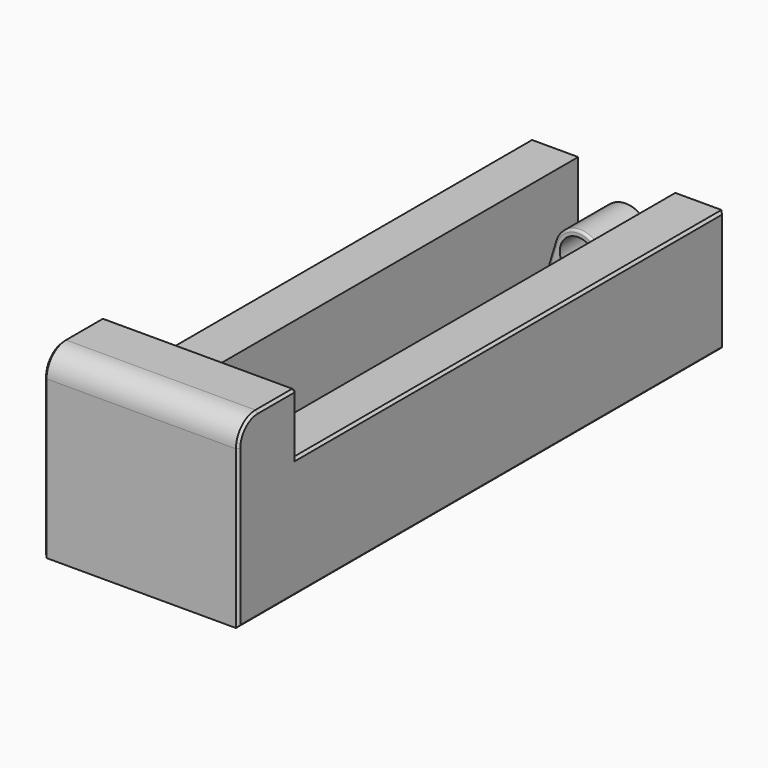
from build123d import *

# Parameters (mm, degrees)
F1_DEPTH = 40
F2_R     = 7.6
F3_DEPTH = 220
F4_DEPTH = 25
F5_SIZE  = 1
F6_R     = 1


with BuildPart() as f1:
    # F0 (on Right) → F1 (new body, symmetric)
    with BuildSketch(Plane.YZ):
        with BuildLine():
            Line((-146.159631235, 0), (0, 0))
            Line((0, 0), (45.9261649855, 0))
            Line((45.9261649855, 0), (103.840368765, 0))
            Line((103.840368765, 0), (103.840368765, 50))
            Line((103.840368765, 50), (-116.159631235, 50))
            Line((-116.159631235, 50), (-116.159631235, 75))
            Line((-116.159631235, 75), (-136.159631235, 75))
            ThreePointArc((-136.159631235, 75), (-143.2306990468, 72.0710678119), (-146.159631235, 65))
            Line((-146.159631235, 65), (-146.159631235, 0))
        make_face()
    extrude(amount=F1_DEPTH, both=True)

    # F2 (on face) → F3 (cut, through all)
    with BuildSketch(Plane(origin=(0, 103.840368765, 0), x_dir=(-1, 0, 0), z_dir=(0, 1, 0))):
        with BuildLine():
            Line((20, 15), (20, 50))
            Line((20, 50), (-20, 50))
            Line((-20, 50), (-20, 15))
            Line((-20, 15), (-15, 15))
            Line((-15, 15), (-9.569428978, 32.9027623113))
            ThreePointArc((-9.569428978, 32.9027623113), (0, 40), (9.569428978, 32.9027623113))
            Line((9.569428978, 32.9027623113), (15, 15))
            Line((15, 15), (20, 15))
        make_face()
        with BuildLine():
            ThreePointArc((10, 30), (9.8917715749, 31.4672610914), (9.569428978, 32.9027623113))
            ThreePointArc((9.569428978, 32.9027623113), (0, 40), (-9.569428978, 32.9027623113))
            ThreePointArc((-9.569428978, 32.9027623113), (-1.4672610914, 20.1082284251), (10, 30))
        make_face()
        with Locations((0, 30)):
            Circle(F2_R, mode=Mode.SUBTRACT)
        with BuildLine():
            Line((-15, 15), (15, 15))
            Line((15, 15), (9.569428978, 32.9027623113))
            ThreePointArc((9.569428978, 32.9027623113), (9.8917715749, 31.4672610914), (10, 30))
            ThreePointArc((10, 30), (-1.4672610914, 20.1082284251), (-9.569428978, 32.9027623113))
            Line((-9.569428978, 32.9027623113), (-15, 15))
        make_face()
        with Locations((0, 30)):
            Circle(F2_R)
    extrude(amount=-F3_DEPTH, mode=Mode.SUBTRACT)

    # F2 (on face) → F4 (join)
    with BuildSketch(Plane(origin=(0, 103.840368765, 0), x_dir=(-1, 0, 0), z_dir=(0, 1, 0))):
        with BuildLine():
            Line((-15, 15), (15, 15))
            Line((15, 15), (9.569428978, 32.9027623113))
            ThreePointArc((9.569428978, 32.9027623113), (9.8917715749, 31.4672610914), (10, 30))
            ThreePointArc((10, 30), (-1.4672610914, 20.1082284251), (-9.569428978, 32.9027623113))
            Line((-9.569428978, 32.9027623113), (-15, 15))
        make_face()
        with BuildLine():
            ThreePointArc((10, 30), (9.8917715749, 31.4672610914), (9.569428978, 32.9027623113))
            ThreePointArc((9.569428978, 32.9027623113), (0, 40), (-9.569428978, 32.9027623113))
            ThreePointArc((-9.569428978, 32.9027623113), (-1.4672610914, 20.1082284251), (10, 30))
        make_face()
        with Locations((0, 30)):
            Circle(F2_R, mode=Mode.SUBTRACT)
    extrude(amount=-F4_DEPTH)

    # F5
    f5_edges = [f1.edges().sort_by_distance(p)[0] for p in [
        (-40, -146.159631, 32.5),
        (-40, -21.159631, 0),
        (-40, 103.840369, 25),
        (-40, -6.159631, 50),
        (-40, -116.159631, 62.5),
        (-40, -126.159631, 75),
        (-40, -143.230699, 72.071068),
        (0, -136.159631, 75),
        (40, -126.159631, 75),
        (0, -116.159631, 75),
        (40, -146.159631, 32.5),
        (40, -21.159631, 0),
        (40, 103.840369, 25),
        (40, -6.159631, 50),
        (40, -116.159631, 62.5),
        (40, -143.230699, 72.071068),
    ]]
    chamfer(f5_edges, length=F5_SIZE)

    # F6
    f6_edges = [f1.edges().sort_by_distance(p)[0] for p in [
        (-12.284714, 103.840369, 23.951381),
        (-15, 91.340369, 15),
        (15, 91.340369, 15),
        (0, 78.840369, 40),
        (-17.5, 103.840369, 15),
        (17.5, 103.840369, 15),
        (12.284714, 103.840369, 23.951381),
        (0, 103.840369, 40),
        (0, 78.840369, 15),
        (-12.284714, 78.840369, 23.951381),
        (12.284714, 78.840369, 23.951381),
    ]]
    fillet(f6_edges, radius=F6_R)


solid = f1.part
